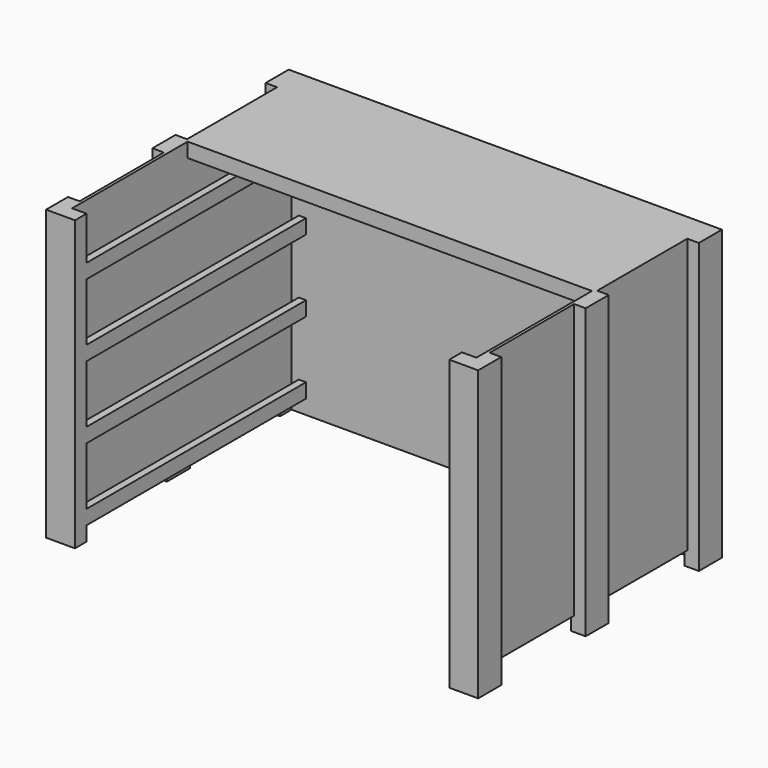
from build123d import *

# Parameters (mm, degrees)
F0_W          = 76.2
F0_H          = 50.8
F1_DEPTH      = 25.4
F1_DEPTH_BACK = 25.4
F2_W          = 71.12
F2_H          = 50.8
F3_DEPTH      = 25.4
F4_W          = 71.12
F4_H          = 48.26
F5_DEPTH      = 22.86
F6_W          = 48.26
F6_H          = 2.54
F7_DEPTH      = 2.54
F8_W          = 48.26
F8_H          = 2.54
F9_DEPTH      = 2.54
F10_W         = 48.26
F10_H         = 2.54
F11_DEPTH     = 2.54
F12_W         = 48.26
F12_H         = 2.54
F13_DEPTH     = 2.54
F15_W         = 1.27
F15_H         = 1.27
F16_DEPTH     = 48.26
F17_W         = 1.27
F17_H         = 1.27
F18_DEPTH     = 48.26
F19_W         = 1.27
F19_H         = 1.2642855102
F20_DEPTH     = 48.26
F21_W         = 1.27
F21_H         = 1.27
F22_DEPTH     = 48.26
F23_W         = 1.27
F23_H         = 1.27
F24_DEPTH     = 48.26
F25_W         = 1.27
F25_H         = 1.27
F26_DEPTH     = 48.26
F27_W         = 1.27
F27_H         = 1.27
F28_DEPTH     = 48.26
F29_W         = 1.27
F29_H         = 1.27
F30_DEPTH     = 48.26
F31_W         = 5.08
F31_H         = 50.8
F32_DEPTH     = 2.794
F33_W         = 5.08
F33_H         = 50.8
F34_DEPTH     = 2.54
F35_W         = 18.5524672455
F35_H         = 50.8
F35_W_2       = 19.8015327545
F36_DEPTH     = 2.032
F37_W         = 18.5524672455
F37_H         = 2.54
F38_DEPTH     = 74.169
F39_W         = 19.8015327545
F39_H         = 2.5402396598
F40_DEPTH     = 74.169


# Not quite as in the source:
# - a pattern or mirror of a feature is missing from the dataset's text; its kind, count and spacing are read off the source's solid


with BuildPart() as f1:
    # F0 (on Front) → F1 (new body, two sides)
    with BuildSketch(Plane.XZ) as f1_sk:
        with Locations((0, 4.3905831537)):
            Rectangle(F0_W, F0_H)
    extrude(amount=F1_DEPTH)
    extrude(f1_sk.sketch, amount=-F1_DEPTH_BACK)

    # F2 (on face) → F3 (cut)
    with BuildSketch(Plane.XZ.offset(25.4)):
        with Locations((0, 4.3905831537)):
            Rectangle(F2_W, F2_H)
    extrude(amount=-F3_DEPTH, mode=Mode.SUBTRACT)

    # F4 (on face) → F5 (cut)
    with BuildSketch(Plane.XZ):
        with Locations((0, 3.1205831537)):
            Rectangle(F4_W, F4_H)
    extrude(amount=-F5_DEPTH, mode=Mode.SUBTRACT)

    # F6 (on face) → F7 (join)
    with BuildSketch(Plane.YZ.offset(-35.56)):
        with Locations((-1.27, -17.1994168463)):
            Rectangle(F6_W, F6_H)
    extrude(amount=F7_DEPTH)

    # F8 (on face) → F9 (join)
    with BuildSketch(Plane.YZ.offset(-35.56)):
        with Locations((-1.27, -4.4994168463)):
            Rectangle(F8_W, F8_H)
    extrude(amount=F9_DEPTH)

    # F10 (on face) → F11 (join)
    with BuildSketch(Plane.YZ.offset(-35.56)):
        with Locations((-1.27, 8.2005831537)):
            Rectangle(F10_W, F10_H)
    extrude(amount=F11_DEPTH)

    # F12 (on face) → F13 (join)
    with BuildSketch(Plane.YZ.offset(-35.56)):
        with Locations((-1.27, 20.9005831537)):
            Rectangle(F12_W, F12_H)
    extrude(amount=F13_DEPTH)

    # F14: F1 across plane


with BuildPart() as f1_1:
    add(f1.part)
    add(f1.part.mirror(Plane.YZ))

    # F15 (on face) → F16 (cut)
    with BuildSketch(Plane.XZ.offset(25.4)):
        with Locations((-34.925, -16.5644168463)):
            Rectangle(F15_W, F15_H)
    extrude(amount=-F16_DEPTH, mode=Mode.SUBTRACT)

    # F17 (on face) → F18 (cut)
    with BuildSketch(Plane.XZ.offset(25.4)):
        with Locations((-34.925, -3.8644168463)):
            Rectangle(F17_W, F17_H)
    extrude(amount=-F18_DEPTH, mode=Mode.SUBTRACT)

    # F19 (on face) → F20 (cut)
    with BuildSketch(Plane.XZ.offset(25.4)):
        with Locations((-34.925, 8.8384403986)):
            Rectangle(F19_W, F19_H)
    extrude(amount=-F20_DEPTH, mode=Mode.SUBTRACT)

    # F21 (on face) → F22 (cut)
    with BuildSketch(Plane.XZ.offset(25.4)):
        with Locations((-34.925, 21.5355831537)):
            Rectangle(F21_W, F21_H)
    extrude(amount=-F22_DEPTH, mode=Mode.SUBTRACT)

    # F23 (on face) → F24 (cut)
    with BuildSketch(Plane.XZ.offset(25.4)):
        with Locations((34.925, 21.5355831537)):
            Rectangle(F23_W, F23_H)
    extrude(amount=-F24_DEPTH, mode=Mode.SUBTRACT)

    # F25 (on face) → F26 (cut)
    with BuildSketch(Plane.XZ.offset(25.4)):
        with Locations((34.925, 8.8355831537)):
            Rectangle(F25_W, F25_H)
    extrude(amount=-F26_DEPTH, mode=Mode.SUBTRACT)

    # F27 (on face) → F28 (cut)
    with BuildSketch(Plane.XZ.offset(25.4)):
        with Locations((34.925, -3.8644168463)):
            Rectangle(F27_W, F27_H)
    extrude(amount=-F28_DEPTH, mode=Mode.SUBTRACT)

    # F29 (on face) → F30 (cut)
    with BuildSketch(Plane.XZ.offset(25.4)):
        with Locations((34.925, -16.5644168463)):
            Rectangle(F29_W, F29_H)
    extrude(amount=-F30_DEPTH, mode=Mode.SUBTRACT)

    # F31 (on face) → F32 (join)
    with BuildSketch(Plane.XZ.offset(25.4)):
        with Locations((35.56, 4.3905831537)):
            Rectangle(F31_W, F31_H)
    extrude(amount=F32_DEPTH)

    # F33 (on face) → F34 (join)
    with BuildSketch(Plane.XZ.offset(25.4)):
        with Locations((-35.56, 4.3905831537)):
            Rectangle(F33_W, F33_H)
    extrude(amount=F34_DEPTH)

    # F35 (on face) → F36 (cut)
    with BuildSketch(Plane.YZ.offset(38.1)):
        with Locations((-13.8377663772, 4.3905831537)):
            Rectangle(F35_W, F35_H)
        with Locations((10.4192336228, 4.3905831537)):
            Rectangle(F35_W_2, F35_H)
    f36 = extrude(amount=-F36_DEPTH, mode=Mode.SUBTRACT)

    # F36_copies: F36 across plane
    add(f36.mirror(Plane(origin=(0, 0, 0), x_dir=(0, 0, -1), z_dir=(-1, 0, 0))), mode=Mode.SUBTRACT)

    # F37 (on face) → F38 (cut, through all)
    with BuildSketch(Plane.YZ.offset(36.068)):
        with Locations((-13.8377663772, -19.7394168463)):
            Rectangle(F37_W, F37_H)
    extrude(amount=-F38_DEPTH, mode=Mode.SUBTRACT)

    # F39 (on face) → F40 (cut, through all)
    with BuildSketch(Plane.YZ.offset(36.068)):
        with Locations((10.4192336228, -19.7392970164)):
            Rectangle(F39_W, F39_H)
    extrude(amount=-F40_DEPTH, mode=Mode.SUBTRACT)


solid = f1_1.part
